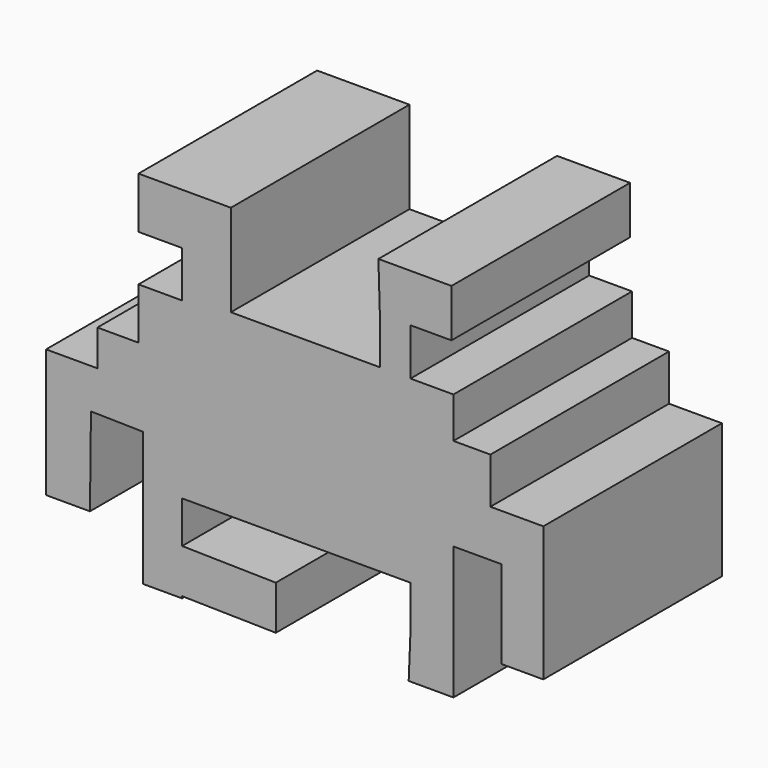
from build123d import *

# Parameters (mm, degrees)
F0_W     = 4.8859491944
F0_H     = 5.7481750846
F0_W_2   = 5.4607708007
F0_W_3   = 4.5850016177
F0_H_2   = 5.367808044
F2_DEPTH = 25
F3_DEPTH = 25
F4_DEPTH = 25
F5_DEPTH = 25


with BuildPart() as f2:
    # F0 (on Front) → F2 (new body)
    with BuildSketch(Plane.XZ):
        Polygon((10.7778282836, 36.3572090864), (10.7778282836, 21.9867695123), (15.6911015511, 21.9867695123), (15.8029310405, 31.8775773048), (17.372814146, 31.8473872064), (21.6180570424, 31.7657478154), (21.6180570424, 21.9247676432), (26.0104928166, 21.9247676432), (26.0104928166, 26.6215987504), (51.5883155167, 26.6215987504), (51.5883155167, 21.9247676432), (56.3969761133, 21.9247676432), (56.3969761133, 31.7657478154), (61.7647841573, 31.7657478154), (61.7647841573, 21.9247676432), (66.4616152644, 21.9247676432), (66.4616152644, 37.0217263699), (61.0938072205, 37.0217263699), (60.5346597731, 37.0217263699), (60.5346597731, 42.1658754349), (56.3969761133, 42.1658754349), (56.3969761133, 46.7486605048), (51.5883155167, 46.7486605048), (51.5883155167, 51.7831966281), (51.5883155167, 52.006855607), (48.1558144093, 52.006855607), (48.1558144093, 46.7486605048), (31.7722000182, 46.7486605048), (31.4712636173, 46.7486605048), (31.4712636173, 51.3024665415), (26.0104928166, 51.3024665415), (26.0104928166, 46.1291074753), (21.1245436221, 46.1291074753), (21.1245436221, 40.380936116), (16.5260042995, 40.380936116), (16.5260042995, 36.3572090864), (11.9274631143, 36.3572090864), align=None)
        Polygon((26.0104928166, 21.9247676432), (21.6180570424, 21.9247676432), (21.6180570424, 21.3656201959), (21.6180570424, 16.7604498565), (26.0104928166, 16.7604498565), (26.0104928166, 16.9814561175), align=None)
        Polygon((36.504591053, 21.7229578032), (26.0104928166, 21.9247676432), (26.0104928166, 16.9814561175), (36.504591053, 16.7796462774), align=None)
        with Locations((23.5675182194, 54.1765540838)):
            Rectangle(F0_W, F0_H)
        with Locations((28.7408782169, 54.1765540838)):
            Rectangle(F0_W_2, F0_H)
        Polygon((56.3969761133, 21.9247676432), (51.5883155167, 21.9247676432), (51.3829626143, 16.872657463), (56.2078505754, 16.872657463), (56.3969761133, 16.872657463), (56.3969761133, 17.3397641629), align=None)
        Polygon((47.9939952493, 57.374663651), (48.1558144093, 52.006855607), (51.5883155167, 52.006855607), (51.5883155167, 57.374663651), align=None)
        with Locations((53.8808163255, 54.690759629)):
            Rectangle(F0_W_3, F0_H_2)
    extrude(amount=F2_DEPTH)


with BuildPart() as f3:
    # F0 (on Front) → F3 (new body)
    with BuildSketch(Plane.XZ):
        Polygon((10.7778282836, 36.3572090864), (10.7778282836, 21.9867695123), (15.6911015511, 21.9867695123), (15.8029310405, 31.8775773048), (17.372814146, 31.8473872064), (21.6180570424, 31.7657478154), (21.6180570424, 21.9247676432), (26.0104928166, 21.9247676432), (26.0104928166, 26.6215987504), (51.5883155167, 26.6215987504), (51.5883155167, 21.9247676432), (56.3969761133, 21.9247676432), (56.3969761133, 31.7657478154), (61.7647841573, 31.7657478154), (61.7647841573, 21.9247676432), (66.4616152644, 21.9247676432), (66.4616152644, 37.0217263699), (61.0938072205, 37.0217263699), (60.5346597731, 37.0217263699), (60.5346597731, 42.1658754349), (56.3969761133, 42.1658754349), (56.3969761133, 46.7486605048), (51.5883155167, 46.7486605048), (51.5883155167, 51.7831966281), (51.5883155167, 52.006855607), (48.1558144093, 52.006855607), (48.1558144093, 46.7486605048), (31.7722000182, 46.7486605048), (31.4712636173, 46.7486605048), (31.4712636173, 51.3024665415), (26.0104928166, 51.3024665415), (26.0104928166, 46.1291074753), (21.1245436221, 46.1291074753), (21.1245436221, 40.380936116), (16.5260042995, 40.380936116), (16.5260042995, 36.3572090864), (11.9274631143, 36.3572090864), align=None)
        Polygon((26.0104928166, 21.9247676432), (21.6180570424, 21.9247676432), (21.6180570424, 21.3656201959), (21.6180570424, 16.7604498565), (26.0104928166, 16.7604498565), (26.0104928166, 16.9814561175), align=None)
        Polygon((36.504591053, 21.7229578032), (26.0104928166, 21.9247676432), (26.0104928166, 16.9814561175), (36.504591053, 16.7796462774), align=None)
        with Locations((23.5675182194, 54.1765540838)):
            Rectangle(F0_W, F0_H)
        with Locations((28.7408782169, 54.1765540838)):
            Rectangle(F0_W_2, F0_H)
        Polygon((56.3969761133, 21.9247676432), (51.5883155167, 21.9247676432), (51.3829626143, 16.872657463), (56.2078505754, 16.872657463), (56.3969761133, 16.872657463), (56.3969761133, 17.3397641629), align=None)
        Polygon((47.9939952493, 57.374663651), (48.1558144093, 52.006855607), (51.5883155167, 52.006855607), (51.5883155167, 57.374663651), align=None)
        with Locations((53.8808163255, 54.690759629)):
            Rectangle(F0_W_3, F0_H_2)
    extrude(amount=F3_DEPTH)


with BuildPart() as f4:
    # F0 (on Front) → F4 (new body)
    with BuildSketch(Plane.XZ):
        Polygon((10.7778282836, 36.3572090864), (10.7778282836, 21.9867695123), (15.6911015511, 21.9867695123), (15.8029310405, 31.8775773048), (17.372814146, 31.8473872064), (21.6180570424, 31.7657478154), (21.6180570424, 21.9247676432), (26.0104928166, 21.9247676432), (26.0104928166, 26.6215987504), (51.5883155167, 26.6215987504), (51.5883155167, 21.9247676432), (56.3969761133, 21.9247676432), (56.3969761133, 31.7657478154), (61.7647841573, 31.7657478154), (61.7647841573, 21.9247676432), (66.4616152644, 21.9247676432), (66.4616152644, 37.0217263699), (61.0938072205, 37.0217263699), (60.5346597731, 37.0217263699), (60.5346597731, 42.1658754349), (56.3969761133, 42.1658754349), (56.3969761133, 46.7486605048), (51.5883155167, 46.7486605048), (51.5883155167, 51.7831966281), (51.5883155167, 52.006855607), (48.1558144093, 52.006855607), (48.1558144093, 46.7486605048), (31.7722000182, 46.7486605048), (31.4712636173, 46.7486605048), (31.4712636173, 51.3024665415), (26.0104928166, 51.3024665415), (26.0104928166, 46.1291074753), (21.1245436221, 46.1291074753), (21.1245436221, 40.380936116), (16.5260042995, 40.380936116), (16.5260042995, 36.3572090864), (11.9274631143, 36.3572090864), align=None)
        Polygon((26.0104928166, 21.9247676432), (21.6180570424, 21.9247676432), (21.6180570424, 21.3656201959), (21.6180570424, 16.7604498565), (26.0104928166, 16.7604498565), (26.0104928166, 16.9814561175), align=None)
        Polygon((36.504591053, 21.7229578032), (26.0104928166, 21.9247676432), (26.0104928166, 16.9814561175), (36.504591053, 16.7796462774), align=None)
        with Locations((23.5675182194, 54.1765540838)):
            Rectangle(F0_W, F0_H)
        with Locations((28.7408782169, 54.1765540838)):
            Rectangle(F0_W_2, F0_H)
        Polygon((56.3969761133, 21.9247676432), (51.5883155167, 21.9247676432), (51.3829626143, 16.872657463), (56.2078505754, 16.872657463), (56.3969761133, 16.872657463), (56.3969761133, 17.3397641629), align=None)
        Polygon((47.9939952493, 57.374663651), (48.1558144093, 52.006855607), (51.5883155167, 52.006855607), (51.5883155167, 57.374663651), align=None)
        with Locations((53.8808163255, 54.690759629)):
            Rectangle(F0_W_3, F0_H_2)
    extrude(amount=F4_DEPTH)


with BuildPart() as f5:
    # F0 (on Front) → F5 (new body)
    with BuildSketch(Plane.XZ):
        Polygon((10.7778282836, 36.3572090864), (10.7778282836, 21.9867695123), (15.6911015511, 21.9867695123), (15.8029310405, 31.8775773048), (17.372814146, 31.8473872064), (21.6180570424, 31.7657478154), (21.6180570424, 21.9247676432), (26.0104928166, 21.9247676432), (26.0104928166, 26.6215987504), (51.5883155167, 26.6215987504), (51.5883155167, 21.9247676432), (56.3969761133, 21.9247676432), (56.3969761133, 31.7657478154), (61.7647841573, 31.7657478154), (61.7647841573, 21.9247676432), (66.4616152644, 21.9247676432), (66.4616152644, 37.0217263699), (61.0938072205, 37.0217263699), (60.5346597731, 37.0217263699), (60.5346597731, 42.1658754349), (56.3969761133, 42.1658754349), (56.3969761133, 46.7486605048), (51.5883155167, 46.7486605048), (51.5883155167, 51.7831966281), (51.5883155167, 52.006855607), (48.1558144093, 52.006855607), (48.1558144093, 46.7486605048), (31.7722000182, 46.7486605048), (31.4712636173, 46.7486605048), (31.4712636173, 51.3024665415), (26.0104928166, 51.3024665415), (26.0104928166, 46.1291074753), (21.1245436221, 46.1291074753), (21.1245436221, 40.380936116), (16.5260042995, 40.380936116), (16.5260042995, 36.3572090864), (11.9274631143, 36.3572090864), align=None)
        Polygon((26.0104928166, 21.9247676432), (21.6180570424, 21.9247676432), (21.6180570424, 21.3656201959), (21.6180570424, 16.7604498565), (26.0104928166, 16.7604498565), (26.0104928166, 16.9814561175), align=None)
        Polygon((36.504591053, 21.7229578032), (26.0104928166, 21.9247676432), (26.0104928166, 16.9814561175), (36.504591053, 16.7796462774), align=None)
        with Locations((23.5675182194, 54.1765540838)):
            Rectangle(F0_W, F0_H)
        with Locations((28.7408782169, 54.1765540838)):
            Rectangle(F0_W_2, F0_H)
        Polygon((56.3969761133, 21.9247676432), (51.5883155167, 21.9247676432), (51.3829626143, 16.872657463), (56.2078505754, 16.872657463), (56.3969761133, 16.872657463), (56.3969761133, 17.3397641629), align=None)
        Polygon((47.9939952493, 57.374663651), (48.1558144093, 52.006855607), (51.5883155167, 52.006855607), (51.5883155167, 57.374663651), align=None)
        with Locations((53.8808163255, 54.690759629)):
            Rectangle(F0_W_3, F0_H_2)
    extrude(amount=F5_DEPTH)


solid = Compound([f2.part, f3.part, f4.part, f5.part])
